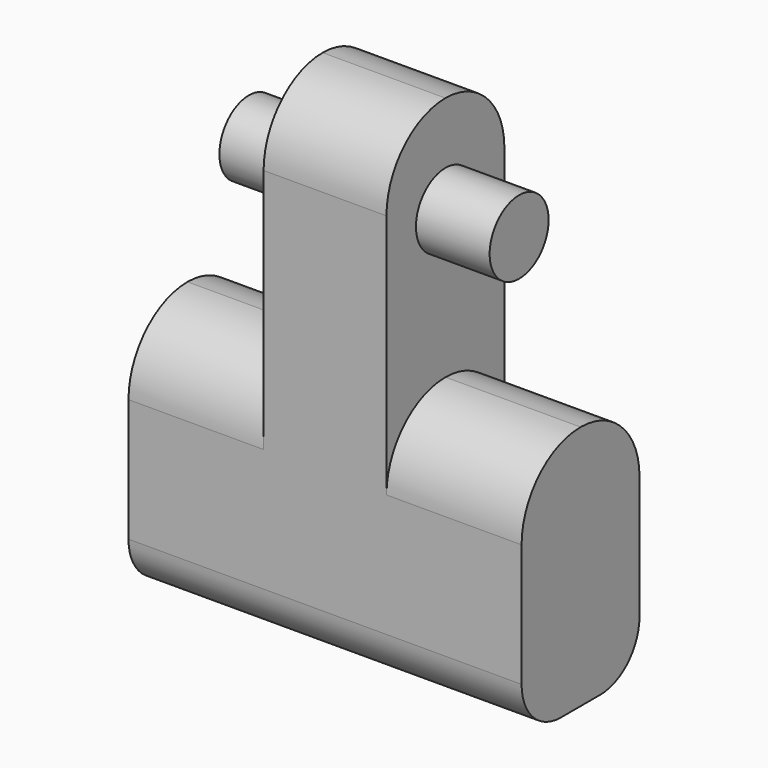
from build123d import *

# Parameters (mm, degrees)
F1_DEPTH      = 6
F2_R          = 1.5
F3_DEPTH      = 3
F3_DEPTH_BACK = 8
F4_R          = 2.99999
F5_R          = 2.99999
F6_R          = 2


# Not quite as in the source:
# - a fillet or chamfer is up to 0.001 mm smaller than in the source, because OpenCascade refuses the exact size


with BuildPart() as f1:
    # F0 (on Front) → F1 (new body)
    with BuildSketch(Plane.XZ):
        Polygon((5.5, 0), (0, 0), (0, -10), (16, -10), (16, 0), (10.5, 0), (10.5, 10), (5.5, 10), align=None)
    extrude(amount=F1_DEPTH)

    # F2 (on face) → F3 (join, two sides)
    with BuildSketch(Plane.YZ.offset(10.5)) as f3_sk:
        with Locations((-3, 6)):
            Circle(F2_R)
    extrude(amount=F3_DEPTH)
    extrude(f3_sk.sketch, amount=-F3_DEPTH_BACK)

    # F4 (radius 3 in the source; OpenCascade refuses exactly that, so slightly less here)
    f4_edges = [f1.edges().sort_by_distance(p)[0] for p in [
        (8, -6, 10),
        (8, 0, 10),
    ]]
    fillet(f4_edges, radius=F4_R)

    # F5 (radius 3 in the source; OpenCascade refuses exactly that, so slightly less here)
    f5_edges = [f1.edges().sort_by_distance(p)[0] for p in [
        (2.75, -6, 0),
        (2.75, 0, 0),
        (13.25, -6, 0),
        (13.25, 0, 0),
    ]]
    fillet(f5_edges, radius=F5_R)

    # F6
    f6_edges = [f1.edges().sort_by_distance(p)[0] for p in [
        (8, -6, -10),
        (8, 0, -10),
    ]]
    fillet(f6_edges, radius=F6_R)


solid = f1.part
